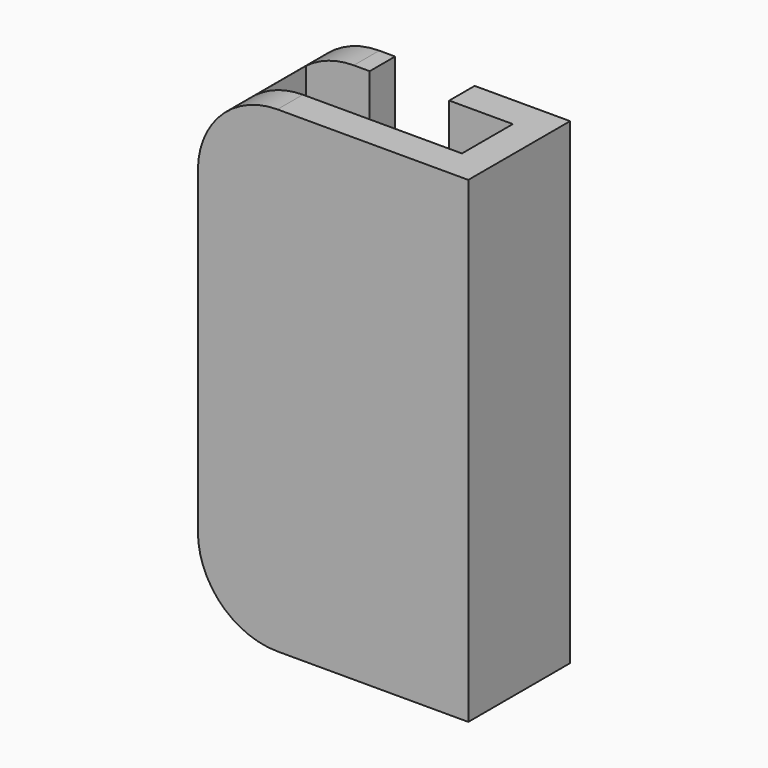
from build123d import *

# Parameters (mm, degrees)
F0_W        = 4
F0_H        = 2
F0_W_2      = 2
F0_H_2      = 4
F0_W_3      = 6.5
F1_DEPTH    = 15
F2_T1_DEPTH = 33


# Not quite as in the source:
# - a fillet or chamfer that OpenCascade refuses, or shapes differently, is made with other operations: its cross-section is extruded or revolved along the edge and cut away or added


with BuildPart() as f1:
    # F0 (on Top) → F1 (new body, symmetric)
    with BuildSketch(Plane.XY):
        with Locations((-4.5, 7)):
            Rectangle(F0_W, F0_H)
        with Locations((-7.5, 7)):
            Rectangle(F0_W_2, F0_H)
        with Locations((-7.5, 4)):
            Rectangle(F0_W_2, F0_H_2)
        with Locations((-7.5, 1)):
            Rectangle(F0_W_2, F0_H)
        with Locations((-3.25, 1)):
            Rectangle(F0_W_3, F0_H)
        with Locations((3.25, 1)):
            Rectangle(F0_W_3, F0_H)
        with Locations((7.5, 1)):
            Rectangle(F0_W_2, F0_H)
        with Locations((7.5, 4)):
            Rectangle(F0_W_2, F0_H_2)
        with Locations((7.5, 7)):
            Rectangle(F0_W_2, F0_H)
        with Locations((4.5, 7)):
            Rectangle(F0_W, F0_H)
    extrude(amount=F1_DEPTH, both=True)

    # F2: fillet of radius 5 on 2 edges, made by hand

    # F2_s2 → F2_t1 (cut)
    with BuildSketch(Plane.XZ.offset(-20.5)):
        with BuildLine():
            ThreePointArc((-8.5, -10), (-7.0355339059, -13.5355339059), (-3.5, -15))
            Line((-3.5, -15), (-8.5, -15))
            Line((-8.5, -15), (-8.5, -10))
        make_face()
        with BuildLine():
            ThreePointArc((-8.5, 10), (-7.0355339059, 13.5355339059), (-3.5, 15))
            Line((-3.5, 15), (-8.5, 15))
            Line((-8.5, 15), (-8.5, 10))
        make_face()
    extrude(amount=F2_T1_DEPTH, mode=Mode.SUBTRACT)


solid = f1.part
